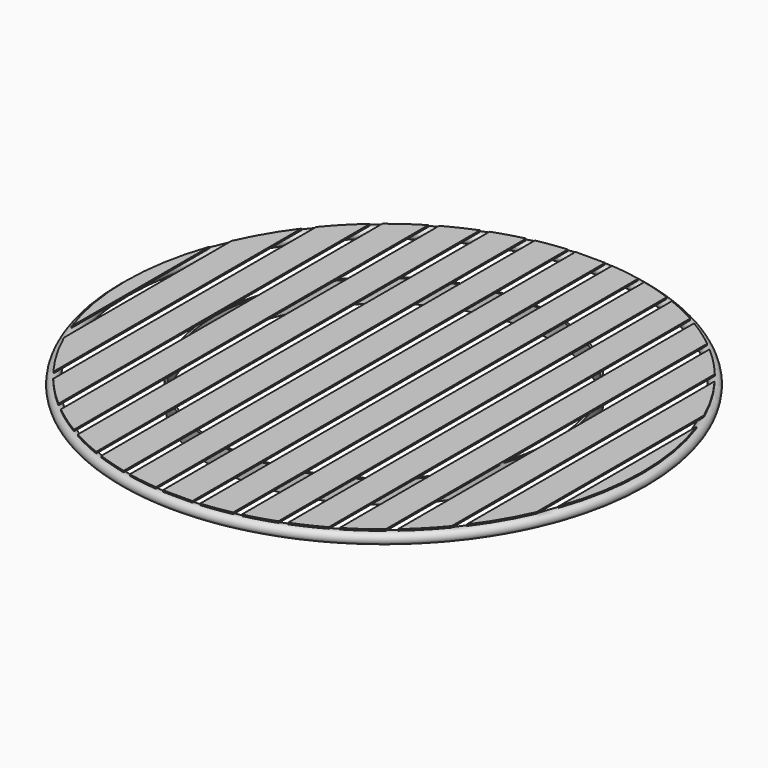
from build123d import *

# Parameters (mm, degrees)
F1_R          = 7.5
F1_R_2        = 5.5
F4_W          = 40
F4_H          = 698.8562083862
F5_DEPTH      = 2
F5_DEPTH_BACK = 0.1
F6_R          = 232
F6_R_2        = 229
F7_DEPTH      = 30


# Not quite as in the source:
# - a feature names something its author has since deleted; it is built from what else it names


with BuildPart() as f2:
    # F2: sweep along a path in F0
    with BuildLine(Plane.XY) as f2_path:
        CenterArc((0, 0), 350, 0, 360)
    # F1 (on Front) → F2 (sweep)
    with BuildSketch(Plane.XZ):
        with Locations((-350, 0)):
            Circle(F1_R)
        with Locations((-350, 0)):
            Circle(F1_R_2, mode=Mode.SUBTRACT)
    sweep(path=f2_path.line)

    # F4 (on offset) → F5 (join, two sides)
    with BuildSketch(Plane.XY.offset(7.5)) as f5_sk:
        with BuildLine():
            Line((-280, -210), (-280, 210))
            ThreePointArc((-280, 210), (-301.9332389408, 177.0206745629), (-320, 141.7744687876))
            Line((-320, 141.7744687876), (-320, -141.7744687876))
            ThreePointArc((-320, -141.7744687876), (-301.9332389408, -177.0206745629), (-280, -210))
        make_face()
        with BuildLine():
            Line((-230, -263.8181191655), (-230, 263.8181191655))
            ThreePointArc((-230, 263.8181191655), (-250.8434921556, 244.0851131125), (-270, 222.7105745132))
            Line((-270, 222.7105745132), (-270, -222.7105745132))
            ThreePointArc((-270, -222.7105745132), (-250.8434921556, -244.0851131125), (-230, -263.8181191655))
        make_face()
        with BuildLine():
            Line((-180, -300.1666203961), (-180, 300.1666203961))
            ThreePointArc((-180, 300.1666203961), (-200.4877779366, 286.8878716468), (-220, 272.2131517763))
            Line((-220, 272.2131517763), (-220, -272.2131517763))
            ThreePointArc((-220, -272.2131517763), (-200.4877779366, -286.8878716468), (-180, -300.1666203961))
        make_face()
        with BuildLine():
            Line((-130, -324.9615361854), (-130, 324.9615361854))
            ThreePointArc((-130, 324.9615361854), (-150.3011762253, 316.0847298199), (-170, 305.9411708156))
            Line((-170, 305.9411708156), (-170, -305.9411708156))
            ThreePointArc((-170, -305.9411708156), (-150.3011762253, -316.0847298199), (-130, -324.9615361854))
        make_face()
        with BuildLine():
            Line((-80, -340.734500748), (-80, 340.734500748))
            ThreePointArc((-80, 340.734500748), (-100.1783099861, 335.3569832407), (-120, 328.7856444555))
            Line((-120, 328.7856444555), (-120, -328.7856444555))
            ThreePointArc((-120, -328.7856444555), (-100.1783099861, -335.3569832407), (-80, -340.734500748))
        make_face()
        with BuildLine():
            Line((-30, -348.7119154833), (-30, 348.7119154833))
            ThreePointArc((-30, 348.7119154833), (-50.0835480834, 346.3980921012), (-70, 342.9285639896))
            Line((-70, 342.9285639896), (-70, -342.9285639896))
            ThreePointArc((-70, -342.9285639896), (-50.0835480834, -346.3980921012), (-30, -348.7119154833))
        make_face()
        Rectangle(F4_W, F4_H)
        with BuildLine():
            Line((-330, -116.6190378969), (-330, 116.6190378969))
            ThreePointArc((-330, 116.6190378969), (-350, 0), (-330, -116.6190378969))
        make_face()
        with BuildLine():
            Line((70, -342.9285639896), (70, 342.9285639896))
            ThreePointArc((70, 342.9285639896), (50.0835480834, 346.3980921012), (30, 348.7119154833))
            Line((30, 348.7119154833), (30, -348.7119154833))
            ThreePointArc((30, -348.7119154833), (50.0835480834, -346.3980921012), (70, -342.9285639896))
        make_face()
        with BuildLine():
            Line((120, -328.7856444555), (120, 328.7856444555))
            ThreePointArc((120, 328.7856444555), (100.1783099861, 335.3569832407), (80, 340.734500748))
            Line((80, 340.734500748), (80, -340.734500748))
            ThreePointArc((80, -340.734500748), (100.1783099861, -335.3569832407), (120, -328.7856444555))
        make_face()
        with BuildLine():
            Line((170, -305.9411708156), (170, 305.9411708156))
            ThreePointArc((170, 305.9411708156), (150.3011762253, 316.0847298199), (130, 324.9615361854))
            Line((130, 324.9615361854), (130, -324.9615361854))
            ThreePointArc((130, -324.9615361854), (150.3011762253, -316.0847298199), (170, -305.9411708156))
        make_face()
        with BuildLine():
            Line((220, -272.2131517763), (220, 272.2131517763))
            ThreePointArc((220, 272.2131517763), (200.4877779366, 286.8878716468), (180, 300.1666203961))
            Line((180, 300.1666203961), (180, -300.1666203961))
            ThreePointArc((180, -300.1666203961), (200.4877779366, -286.8878716468), (220, -272.2131517763))
        make_face()
        with BuildLine():
            Line((270, -222.7105745132), (270, 222.7105745132))
            ThreePointArc((270, 222.7105745132), (250.8434921556, 244.0851131125), (230, 263.8181191655))
            Line((230, 263.8181191655), (230, -263.8181191655))
            ThreePointArc((230, -263.8181191655), (250.8434921556, -244.0851131125), (270, -222.7105745132))
        make_face()
        with BuildLine():
            ThreePointArc((330, -116.6190378969), (344.9637662132, -59.160797831), (350, 0))
            ThreePointArc((350, 0), (344.9637662132, 59.160797831), (330, 116.6190378969))
            Line((330, 116.6190378969), (330, -116.6190378969))
        make_face()
        with BuildLine():
            Line((320, -141.7744687876), (320, 141.7744687876))
            ThreePointArc((320, 141.7744687876), (301.9332389408, 177.0206745629), (280, 210))
            Line((280, 210), (280, -210))
            ThreePointArc((280, -210), (301.9332389408, -177.0206745629), (320, -141.7744687876))
        make_face()
    extrude(amount=F5_DEPTH)
    extrude(f5_sk.sketch, amount=-F5_DEPTH_BACK)

    # F6 (on face) → F7 (join)
    with BuildSketch(Plane(origin=(0, 0, 7.4), x_dir=(1, 0, 0), z_dir=(0, 0, -1))):
        Circle(F6_R)
        Circle(F6_R_2, mode=Mode.SUBTRACT)
    extrude(amount=F7_DEPTH)


solid = f2.part
